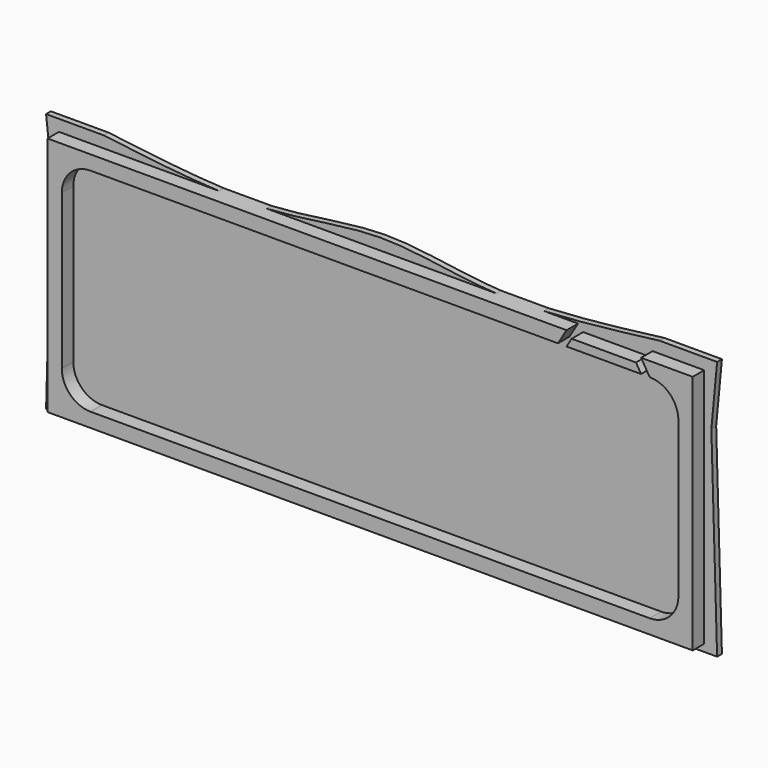
from build123d import *

# Parameters (mm, degrees)
F0_W     = 584.2
F0_H     = 219.71
F1_DEPTH = 5.334
F2_W     = 571.5
F2_H     = 213.36
F2_W_2   = 546.1
F2_H_2   = 187.96
F3_DEPTH = 12.7
F4_R     = 25.4
F6_DEPTH = 12.7
F8_DEPTH = 5.334


# Not quite as in the source:
# - a feature names something its author has since deleted; it is built from what else it names


with BuildPart() as f1:
    # F0 (on Front) → F1 (new body)
    with BuildSketch(Plane.XZ):
        with Locations((-292.1, 109.855)):
            Rectangle(F0_W, F0_H)
    extrude(amount=F1_DEPTH)

    # F2 (on face) → F3 (join)
    with BuildSketch(Plane.XZ.offset(5.334)):
        with Locations((-292.1, 113.03)):
            Rectangle(F2_W, F2_H)
        with Locations((-292.1, 113.03)):
            Rectangle(F2_W_2, F2_H_2, mode=Mode.SUBTRACT)
    extrude(amount=F3_DEPTH)

    # F4
    f4_edges = [f1.edges().sort_by_distance(p)[0] for p in [
        (-565.15, -11.684, 207.01),
        (-19.05, -11.684, 207.01),
        (-19.05, -11.684, 19.05),
        (-565.15, -11.684, 19.05),
    ]]
    fillet(f4_edges, radius=F4_R)

    # F5 (on face) → F6 (cut)
    with BuildSketch(Plane.XZ.offset(18.034)):
        Polygon((-118.11, 219.71), (-125.73, 207.01), (-118.11, 207.01), (-113.5820166854, 214.5566388576), (-110.49, 219.71), align=None)
        Polygon((-56.5979833146, 214.5566388576), (-52.07, 207.01), (-44.45, 207.01), (-52.07, 219.71), (-59.69, 219.71), align=None)
        Polygon((-59.69, 219.71), (-110.49, 219.71), (-113.5820166854, 214.5566388576), (-56.5979833146, 214.5566388576), align=None)
    extrude(amount=-F6_DEPTH, mode=Mode.SUBTRACT)

    # F7 (on face) → F8 (join)
    with BuildSketch(Plane(origin=(0, 0, 0), x_dir=(-1, 0, 0), z_dir=(0, 1, 0))):
        with BuildLine():
            Line((-5.08, 229.87), (0, 176.1275827885))
            Line((0, 176.1275827885), (0, 219.71))
            Line((0, 219.71), (148.0852009026, 219.71))
            add(Edge.make_bspline(
                [(148.0852009026, 219.71), (115.3779899576, 221.1840971885), (80.5489949788, 225.5270485943), (45.72, 229.87)],
                knots=[0.812101374, 0.812101374, 0.812101374, 0.812101374, 1, 1, 1, 1], degree=3))
            Line((45.72, 229.87), (-5.08, 229.87))
        make_face()
        with BuildLine():
            add(Edge.make_bspline(
                [(393.7, 219.71), (356.8171998762, 221.731425099), (324.4585999381, 229.87), (292.1, 229.87)],
                knots=[0.2719218593, 0.2719218593, 0.2719218593, 0.2719218593, 0.5, 0.5, 0.5, 0.5], degree=3))
            add(Edge.make_bspline(
                [(292.1, 229.87), (259.7414000619, 229.87), (227.3828001238, 221.731425099), (190.5, 219.71)],
                knots=[0.5, 0.5, 0.5, 0.5, 0.7280781407, 0.7280781407, 0.7280781407, 0.7280781407], degree=3))
            Line((190.5, 219.71), (393.7, 219.71))
        make_face()
        Polygon((584.2, 183.2547038794), (584.2, 0), (589.28, 0), align=None)
        with BuildLine():
            Line((584.2, 219.71), (584.2, 183.2547038794))
            Line((584.2, 183.2547038794), (589.28, 229.87))
            Line((589.28, 229.87), (538.48, 229.87))
            add(Edge.make_bspline(
                [(538.48, 229.87), (503.6510050212, 225.5270485943), (468.8220100424, 221.1840971885), (436.1147990974, 219.71)],
                knots=[0, 0, 0, 0, 0.187898626, 0.187898626, 0.187898626, 0.187898626], degree=3))
            Line((436.1147990974, 219.71), (584.2, 219.71))
        make_face()
        Polygon((-5.08, 0), (0, 0), (0, 176.1275827885), align=None)
    extrude(amount=-F8_DEPTH)


solid = f1.part
